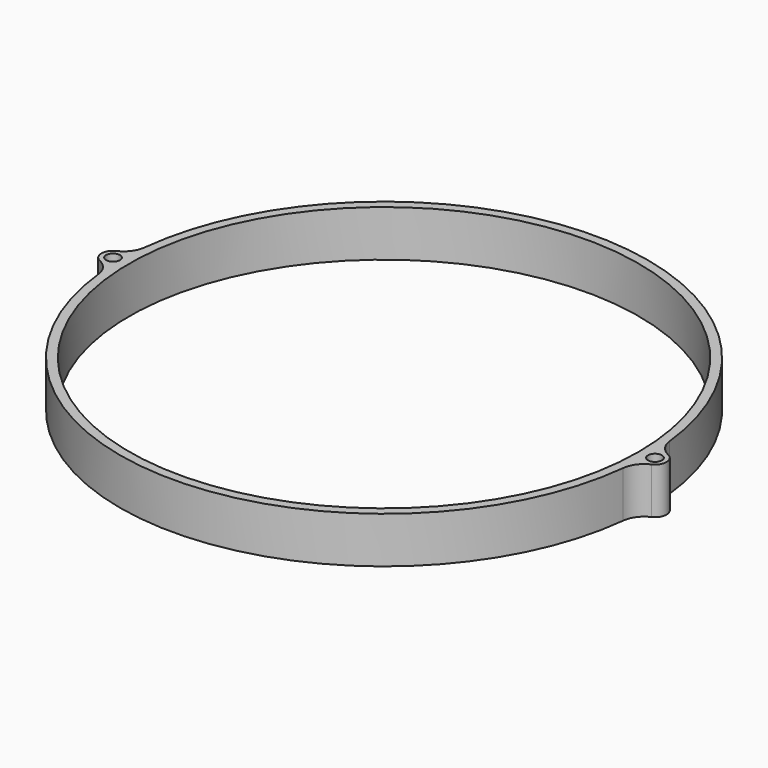
from build123d import *

# Parameters (mm, degrees)
F0_R     = 57
F1_DEPTH = 10
F2_R     = 55
F3_DEPTH = 25
F4_R     = 2.5
F4_R_2   = 1.5
F5_DEPTH = 10
F6_R     = 5


# Not quite as in the source:
# - a pattern or mirror of a feature is missing from the dataset's text; its kind, count and spacing are read off the source's solid


with BuildPart() as f1:
    # F0 (on Top) → F1 (new body)
    with BuildSketch(Plane.XY):
        Circle(F0_R)
    extrude(amount=F1_DEPTH)

    # F2 (on face) → F3 (cut)
    with BuildSketch(Plane.XY.offset(10)):
        Circle(F2_R)
    extrude(amount=-F3_DEPTH, mode=Mode.SUBTRACT)

    # F4 (on Top) → F5 (join)
    with BuildSketch(Plane.XY):
        with Locations((-58.5, 0)):
            Circle(F4_R)
        with Locations((-58.5, 0)):
            Circle(F4_R_2, mode=Mode.SUBTRACT)
    f5 = extrude(amount=F5_DEPTH)

    # F5_copies: F5 across plane
    add(f5.mirror(Plane(origin=(0, 0, 0), x_dir=(0, 0, 1), z_dir=(1, 0, 0))))

    # F6
    f6_edges = [f1.edges().sort_by_distance(p)[0] for p in [
        (-56.965812, 1.973896, 5),
        (-56.965812, -1.973896, 5),
        (56.965812, 1.973896, 5),
        (56.965812, -1.973896, 5),
    ]]
    fillet(f6_edges, radius=F6_R)


solid = f1.part
